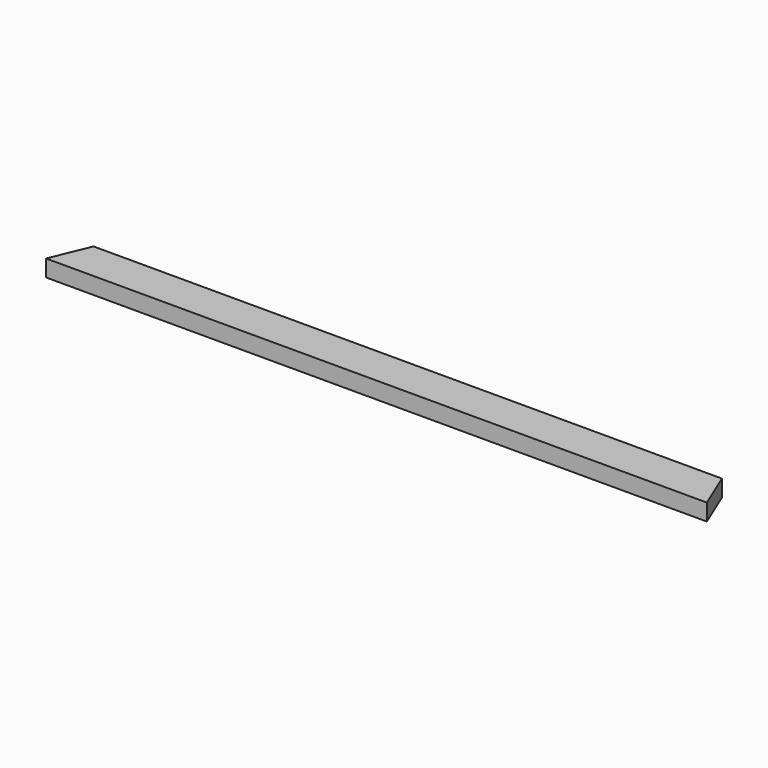
from build123d import *

# Parameters (mm, degrees)
F0_W       = 1503.5709958742
F0_H       = 88.9
F1_DEPTH   = 38.1
F2_SIZE2   = 36.823576
F2_SIZE    = 88.89999
F2_2_SIZE2 = 36.823576
F2_2_SIZE  = 88.89999


# Not quite as in the source:
# - a fillet or chamfer is up to 0.001 mm smaller than in the source, because OpenCascade refuses the exact size


with BuildPart() as f1:
    # F0 (on Top) → F1 (new body)
    with BuildSketch(Plane.XY):
        with Locations((751.7854979371, 44.45)):
            Rectangle(F0_W, F0_H)
    extrude(amount=F1_DEPTH)

    # F2 (size 88.9 and 36.823585695 in the source; OpenCascade refuses exactly that, so slightly less here)
    f2_edges = [f1.edges().sort_by_distance(p)[0] for p in [
        (1503.570996, 88.9, 19.05),
    ]]
    f2_side = f1.faces().sort_by_distance((1503.570996, 44.45, 19.05))[0]
    chamfer(f2_edges, length=F2_SIZE, length2=F2_SIZE2, reference=f2_side)

    # F2#2 (size 88.9 and 36.823585695 in the source; OpenCascade refuses exactly that, so slightly less here)
    f2_2_edges = [f1.edges().sort_by_distance(p)[0] for p in [
        (0, 88.9, 19.05),
    ]]
    f2_2_side = f1.faces().sort_by_distance((0, 44.45, 19.05))[0]
    chamfer(f2_2_edges, length=F2_2_SIZE, length2=F2_2_SIZE2, reference=f2_2_side)


solid = f1.part
